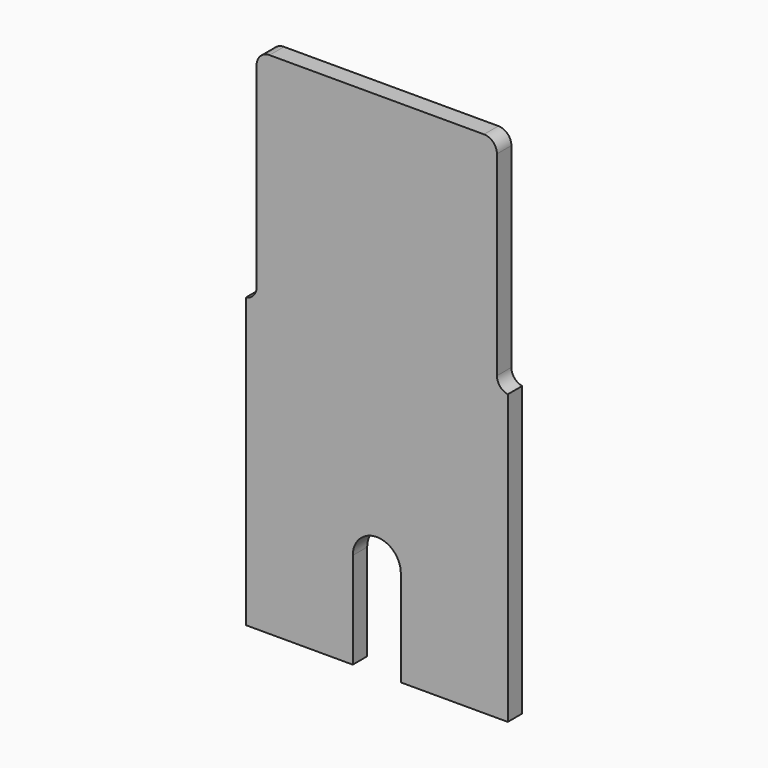
from build123d import *

# Parameters (mm, degrees)
F1_DEPTH    = 9.525
F3_DEPTH    = 25.4
F4_W        = 9.525
F4_H        = 152.4033595958
F5_DEPTH    = 9.525
F6_T1_DEPTH = 9.525


# Not quite as in the source:
# - a fillet or chamfer that OpenCascade refuses, or shapes differently, is made with other operations: its cross-section is extruded or revolved along the edge and cut away or added


with BuildPart() as f1:
    # F0 (on Front) → F1 (new body)
    with BuildSketch(Plane.XZ):
        with BuildLine():
            Line((0, 152.4033595958), (0, 0))
            Line((0, 0), (119.38, 0))
            Line((119.38, 0), (119.38, 152.4033595958))
            ThreePointArc((119.38, 152.4033595958), (122.160179304, 154.9323166344), (123.19, 158.5468))
            Line((123.19, 158.5468), (123.19, 262.382))
            ThreePointArc((123.19, 262.382), (121.1813383054, 267.2313383054), (116.332, 269.24))
            Line((116.332, 269.24), (3.048, 269.24))
            ThreePointArc((3.048, 269.24), (-1.8013383054, 267.2313383054), (-3.81, 262.382))
            Line((-3.81, 262.382), (-3.81, 158.5468))
            ThreePointArc((-3.81, 158.5468), (-2.780179304, 154.9323166344), (0, 152.4033595958))
        make_face()
    extrude(amount=F1_DEPTH)

    # F2 (on face) → F3 (cut)
    with BuildSketch(Plane.XZ.offset(9.525)):
        with BuildLine():
            Line((46.99, 50.8), (46.99, 0))
            Line((46.99, 0), (72.39, 0))
            Line((72.39, 0), (72.39, 50.8))
            ThreePointArc((72.39, 50.8), (59.69, 63.5), (46.99, 50.8))
        make_face()
    extrude(amount=-F3_DEPTH, mode=Mode.SUBTRACT)

    # F4 (on face) → F5 (join)
    with BuildSketch(Plane.XZ.offset(9.525)):
        with Locations((124.1425, 76.2016797979)):
            Rectangle(F4_W, F4_H)
        with Locations((-4.7625, 76.2016797979)):
            Rectangle(F4_W, F4_H)
    extrude(amount=-F5_DEPTH)

    # F6: fillet of radius 6.858 on 2 edges, made by hand

    # F6_s2 → F6_t1 (join)
    with BuildSketch(Plane.XZ):
        with BuildLine():
            ThreePointArc((123.19, 159.1654387879), (124.8101159807, 154.7386188232), (128.905, 152.4033595958))
            Line((128.905, 152.4033595958), (128.7907, 151.7271516766))
            ThreePointArc((128.7907, 151.7271516766), (124.1425, 151.7175595958), (119.38, 151.7175595958))
            Line((119.38, 151.7175595958), (119.0752, 153.0177036362))
            ThreePointArc((119.0752, 153.0177036362), (122.5042, 158.5468), (122.5042, 159.1654387879))
            Line((122.5042, 159.1654387879), (123.19, 159.1654387879))
        make_face()
        with BuildLine():
            ThreePointArc((-9.525, 152.4033595958), (-5.4301159807, 154.7386188232), (-3.81, 159.1654387879))
            Line((-3.81, 159.1654387879), (-3.1242, 159.1654387879))
            ThreePointArc((-3.1242, 159.1654387879), (-3.1242, 158.5468), (0.3048, 153.0177036362))
            Line((0.3048, 153.0177036362), (0, 151.7175595958))
            ThreePointArc((0, 151.7175595958), (-4.7625, 151.7175595958), (-9.4107, 151.7271516766))
            Line((-9.4107, 151.7271516766), (-9.525, 152.4033595958))
        make_face()
    extrude(amount=F6_T1_DEPTH)


solid = f1.part
